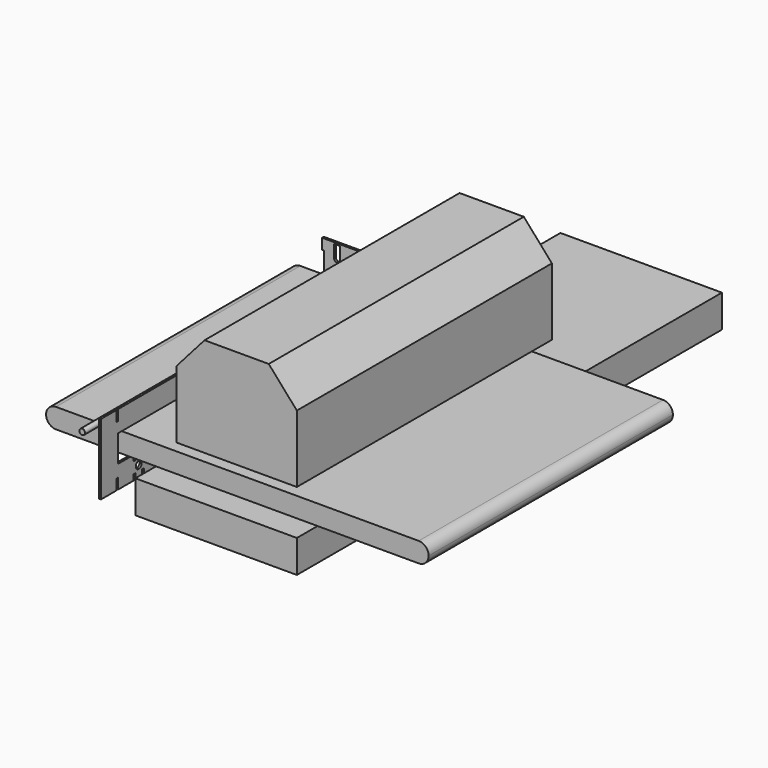
from build123d import *

# Parameters (mm, degrees)
F0_W           = 540
F0_H           = 28
F1_DEPTH       = 431
F2_R           = 13.99999
F3_W           = 228
F3_H           = 46
F4_DEPTH       = 715
F4_DEPTH_BACK  = 35
F6_DEPTH       = 450
F7_R           = 12.5
F7_R_2         = 6
F8_DEPTH       = 400
F9_T           = -5
F10_R          = 5
F11_DEPTH      = 5
F12_R          = 16
F12_R_2        = 5
F13_DEPTH      = 40
F14_R          = 5.25
F15_DEPTH      = 3
F16_W          = 60
F16_H          = 100
F16_R          = 3.5
F16_R_2        = 4.3147526279
F16_R_3        = 5.25
F16_R_4        = 4.483075575
F17_DEPTH      = 3
F18_R          = 5.25
F18_R_2        = 4.25
F19_DEPTH      = 540
F19_DEPTH_BACK = 20
F21_DEPTH      = 3
F22_R          = 4
F23_DEPTH      = 500
F25_DEPTH      = 3


# Not quite as in the source:
# - a fillet or chamfer is up to 0.001 mm smaller than in the source, because OpenCascade refuses the exact size


with BuildPart() as f1:
    # F0 (on Front) → F1 (new body)
    with BuildSketch(Plane.XZ):
        Rectangle(F0_W, F0_H)
    extrude(amount=-F1_DEPTH)

    # F2 (radius 14 in the source; OpenCascade refuses exactly that, so slightly less here)
    f2_edges = [f1.edges().sort_by_distance(p)[0] for p in [
        (-270, 215.5, 14),
        (-270, 215.5, -14),
        (270, 215.5, 14),
        (270, 215.5, -14),
    ]]
    fillet(f2_edges, radius=F2_R)


with BuildPart() as f4:
    # F3 (on face) → F4 (new body, two sides)
    with BuildSketch(Plane.XZ) as f4_sk:
        with Locations((-2, -38)):
            Rectangle(F3_W, F3_H)
    extrude(amount=-F4_DEPTH)
    extrude(f4_sk.sketch, amount=F4_DEPTH_BACK)

    # F9
    f9_openings = [f4.faces().sort_by_distance(p)[0] for p in [
        (-2, 340, -61),
    ]]
    offset(amount=F9_T, openings=f9_openings)

    # F10 (on face) → F11 (cut)
    with BuildSketch(Plane(origin=(-116, 0, 0), x_dir=(0, -1, 0), z_dir=(-1, 0, 0))):
        with Locations((-21, -34)):
            Circle(F10_R)
        with Locations((-408, -34)):
            Circle(F10_R)
    extrude(amount=-F11_DEPTH, mode=Mode.SUBTRACT)


with BuildPart() as f6:
    # F5 (on Front) → F6 (new body)
    with BuildSketch(Plane.XZ):
        Polygon((44.313730334, 165), (-46.313730334, 165), (-86, 120), (-86, 25), (84, 25), (84, 120), align=None)
    extrude(amount=-F6_DEPTH)


with BuildPart() as f8:
    # F7 (on face) → F8 (new body)
    with BuildSketch(Plane.XZ):
        with Locations((-112.0508164167, 32.2285704315)):
            Circle(F7_R)
        with Locations((-112.0508164167, 32.2285704315)):
            Circle(F7_R_2, mode=Mode.SUBTRACT)
    extrude(amount=-F8_DEPTH)


with BuildPart() as f13:
    # F12 (on face) → F13 (new body)
    with BuildSketch(Plane(origin=(-116, 0, 0), x_dir=(0, -1, 0), z_dir=(-1, 0, 0))):
        with Locations((-408, -34)):
            Circle(F12_R)
        with Locations((-408, -34)):
            Circle(F12_R_2, mode=Mode.SUBTRACT)
    extrude(amount=F13_DEPTH)


with BuildPart() as f15:
    # F14 (on face) → F15 (new body)
    with BuildSketch(Plane(origin=(-156, 0, 0), x_dir=(0, -1, 0), z_dir=(-1, 0, 0))):
        with BuildLine():
            Line((-30, -18), (-214.5, -18))
            Line((-214.5, -18), (-399, -18))
            Line((-399, -18), (-399, -20.7712434447))
            ThreePointArc((-399, -20.7712434447), (-393.8578643763, -26.5166852265), (-392, -34))
            ThreePointArc((-392, -34), (-393.8578643763, -41.4833147735), (-399, -47.2287565553))
            Line((-399, -47.2287565553), (-399, -50))
            Line((-399, -50), (-214.5, -50))
            Line((-214.5, -50), (-30, -50))
            Line((-30, -50), (-30, -42))
            Line((-30, -42), (-27, -42))
            Line((-27, -42), (-27, -50))
            Line((-27, -50), (-15, -50))
            Line((-15, -50), (-15, -42))
            Line((-15, -42), (-12, -42))
            Line((-12, -42), (-12, -50))
            Line((-12, -50), (15.5, -50))
            Line((15.5, -50), (15.5, -35))
            Line((15.5, -35), (18.5499999982, -35.0001049883))
            Line((18.5499999982, -35.0001049883), (18.5499999982, -50))
            Line((18.5499999982, -50), (45.5499999982, -50))
            Line((45.5499999982, -50), (45.5499999982, 50))
            Line((45.5499999982, 50), (18.5499999982, 50))
            Line((18.5499999982, 50), (18.5499999982, 35))
            Line((18.5499999982, 35), (15.4999999982, 35))
            Line((15.4999999982, 35), (15.4999999982, 50))
            Line((15.4999999982, 50), (-444.4999999982, 50))
            Line((-444.4999999982, 50), (-444.4999999982, 35))
            Line((-444.4999999982, 35), (-447.5499999982, 35))
            Line((-447.5499999982, 35), (-447.5499999982, 50))
            Line((-447.5499999982, 50), (-474.5499999982, 50))
            Line((-474.5499999982, 50), (-474.5499999982, -50))
            Line((-474.5499999982, -50), (-447.5499999982, -50))
            Line((-447.5499999982, -50), (-447.5499999982, -35))
            Line((-447.5499999982, -35), (-444.4999999982, -35))
            Line((-444.4999999982, -35), (-444.4999999982, -50))
            Line((-444.4999999982, -50), (-417, -50))
            Line((-417, -50), (-417, -47.2287565553))
            ThreePointArc((-417, -47.2287565553), (-424, -34), (-417, -20.7712434447))
            Line((-417, -20.7712434447), (-417, -18))
            Line((-417, -18), (-444.5, -18))
            Line((-444.5, -18), (-444.5, 20))
            Line((-444.5, 20), (15.5, 20))
            Line((15.5, 20), (15.5, -18))
            Line((15.5, -18), (-12, -18))
            Line((-12, -18), (-12, -26))
            Line((-12, -26), (-15, -26))
            Line((-15, -26), (-15, -18))
            Line((-15, -18), (-27, -18))
            Line((-27, -18), (-27, -26))
            Line((-27, -26), (-30, -26))
            Line((-30, -26), (-30, -18))
        make_face()
        with Locations((-21, -34)):
            Circle(F14_R, mode=Mode.SUBTRACT)
        Polygon((-399, -50), (-214.5, -50), (-30, -50), (-30, -42), (-27, -42), (-27, -50), (-15, -50), (-15, -42), (-12, -42), (-12, -50), (15.5, -50), (15.5, -35), (18.5499999982, -35.0001049883), (18.5499999982, -50), (45.5499999982, -50), (45.5499999982, 50), (18.5499999982, 50), (18.5499999982, 35), (15.4999999982, 35), (15.4999999982, 50), (-444.4999999982, 50), (-444.4999999982, 35), (-447.5499999982, 35), (-447.5499999982, 50), (-474.5499999982, 50), (-474.5499999982, -50), (-447.5499999982, -50), (-447.5499999982, -35), (-444.4999999982, -35), (-444.4999999982, -50), (-417, -50), (-417, -42), (-414, -42), (-414, -50), (-402, -50), (-402, -42), (-399, -42), align=None)
        with Locations((-408, -34)):
            Circle(F14_R, mode=Mode.SUBTRACT)
        Polygon((-30, -18), (-214.5, -18), (-399, -18), (-399, -26), (-402, -26), (-402, -18), (-414, -18), (-414, -26), (-417, -26), (-417, -18), (-444.5, -18), (-444.5, 20), (15.5, 20), (15.5, -18), (-12, -18), (-12, -26), (-15, -26), (-15, -18), (-27, -18), (-27, -26), (-30, -26), align=None, mode=Mode.SUBTRACT)
        with Locations((-21, -34)):
            Circle(F14_R, mode=Mode.SUBTRACT)
    extrude(amount=F15_DEPTH)


with BuildPart() as f17:
    # F16 (on face) → F17 (new body)
    with BuildSketch(Plane(origin=(0, 474.5499999982, 0), x_dir=(-1, 0, 0), z_dir=(0, 1, 0))):
        with Locations((186, -100)):
            Rectangle(F16_W, F16_H)
        with Locations((171, -120)):
            Circle(F16_R, mode=Mode.SUBTRACT)
        with Locations((201, -120)):
            Circle(F16_R, mode=Mode.SUBTRACT)
        with Locations((171, -70.4598784447)):
            Circle(F16_R_2, mode=Mode.SUBTRACT)
        with Locations((186, -60)):
            Circle(F16_R_3, mode=Mode.SUBTRACT)
        with Locations((201, -70.4598784447)):
            Circle(F16_R_4, mode=Mode.SUBTRACT)
    extrude(amount=F17_DEPTH)


with BuildPart() as f19:
    # F18 (on face) → F19 (new body, two sides)
    with BuildSketch(Plane.XZ.offset(-474.5499999982)) as f19_sk:
        with Locations((-186, -60)):
            Circle(F18_R)
        with Locations((-186, -60)):
            Circle(F18_R_2, mode=Mode.SUBTRACT)
    extrude(amount=F19_DEPTH)
    extrude(f19_sk.sketch, amount=-F19_DEPTH_BACK)


with BuildPart() as f21:
    # F20 (on face) → F21 (new body)
    with BuildSketch(Plane(origin=(0, 444.4999999982, 0), x_dir=(-1, 0, 0), z_dir=(0, 1, 0))):
        Polygon((236, 50), (156, 50), (156, 35), (159, 35), (159, -35), (156, -35), (156, -50), (236, -50), (236, -35), (233, -35), (233, 35), (236, 35), align=None)
        with BuildLine():
            Line((179, -5), (179, -30))
            ThreePointArc((179, -30), (177, -32), (175, -30))
            Line((175, -30), (175, -5))
            ThreePointArc((175, -5), (177, -3), (179, -5))
        make_face(mode=Mode.SUBTRACT)
        with BuildLine():
            Line((221, -5), (221, -30))
            ThreePointArc((221, -30), (219, -32), (217, -30))
            Line((217, -30), (217, -5))
            ThreePointArc((217, -5), (219, -3), (221, -5))
        make_face(mode=Mode.SUBTRACT)
        with BuildLine():
            Line((172.975, 30), (172.975, 48))
            Line((172.975, 48), (181.025, 48))
            Line((181.025, 48), (181.025, 30))
            ThreePointArc((181.025, 30), (177, 25.975), (172.975, 30))
        make_face(mode=Mode.SUBTRACT)
        with BuildLine():
            Line((210.975, 30), (210.975, 48))
            Line((210.975, 48), (219.025, 48))
            Line((219.025, 48), (219.025, 30))
            ThreePointArc((219.025, 30), (215, 25.975), (210.975, 30))
        make_face(mode=Mode.SUBTRACT)
    extrude(amount=F21_DEPTH)


with BuildPart() as f23:
    # F22 (on face) → F23 (new body)
    with BuildSketch(Plane(origin=(0, 447.4999999982, 0), x_dir=(-1, 0, 0), z_dir=(0, 1, 0))):
        with Locations((177, 30)):
            Circle(F22_R)
    extrude(amount=-F23_DEPTH)


with BuildPart() as f25:
    # F24 (on face) → F25 (new body)
    with BuildSketch(Plane(origin=(0, 414, 0), x_dir=(-1, 0, 0), z_dir=(0, 1, 0))):
        Polygon((239, -18), (159, -18), (159, -26), (162, -26), (162, -42), (159.0808033943, -42), (159.0808033943, -50), (239, -50), (239, -42), (236, -42), (236, -26), (239, -26), align=None)
    extrude(amount=F25_DEPTH)


solid = Compound([f1.part, f4.part, f6.part, f13.part, f15.part, f17.part, f21.part, f23.part, f25.part])
